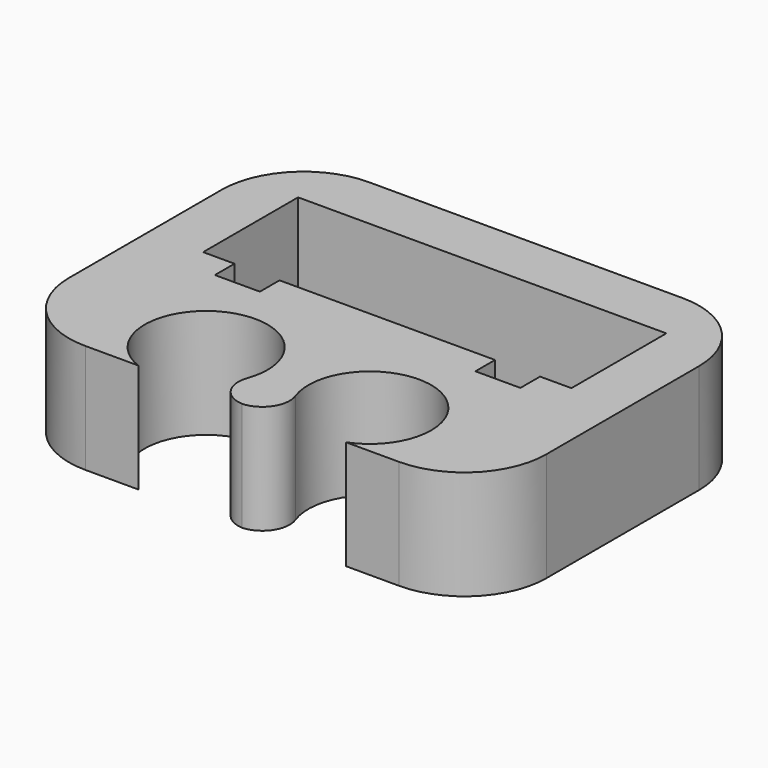
from build123d import *

# Parameters (mm, degrees)
F1_DEPTH    = 4
F2_R        = 3
F3_T1_DEPTH = 15.252055078


# Not quite as in the source:
# - a fillet or chamfer that OpenCascade refuses, or shapes differently, is made with other operations: its cross-section is extruded or revolved along the edge and cut away or added


with BuildPart() as f1:
    # F0 (on Top) → F1 (new body)
    with BuildSketch(Plane.XY):
        with BuildLine():
            Line((8.75, 4.175), (-8.75, 4.175))
            Line((-8.75, 4.175), (-8.75, -8.825))
            Line((-8.75, -8.825), (-3.8077747211, -8.825))
            ThreePointArc((-3.8077747211, -8.825), (-4.2737752701, -4.8702772279), (-0.75, -6.725))
            ThreePointArc((-0.75, -6.725), (-1.1452772279, -7.9987752701), (-2.1922252789, -8.825))
            Line((-2.1922252789, -8.825), (2.1922252789, -8.825))
            ThreePointArc((2.1922252789, -8.825), (1.7262247299, -4.8702772279), (5.25, -6.725))
            ThreePointArc((5.25, -6.725), (4.8547227721, -7.9987752701), (3.8077747211, -8.825))
            Line((3.8077747211, -8.825), (8.75, -8.825))
            Line((8.75, -8.825), (8.75, 4.175))
        make_face()
        Polygon((-6.75, 2.175), (6.75, 2.175), (6.75, -2.175), (5.6, -2.175), (5.6, -3.075), (3.95, -3.075), (3.95, -2.175), (-3.95, -2.175), (-3.95, -3.075), (-5.6, -3.075), (-5.6, -2.175), (-6.75, -2.175), align=None, mode=Mode.SUBTRACT)
    extrude(amount=F1_DEPTH)

    # F2
    f2_edges = [f1.edges().sort_by_distance(p)[0] for p in [
        (-8.75, 4.175, 2),
        (-8.75, -8.825, 2),
        (8.75, -8.825, 2),
        (8.75, 4.175, 2),
    ]]
    fillet(f2_edges, radius=F2_R)

    # F3: fillet of radius 1 on 2 edges, made by hand

    # F3_s2 → F3_t1 (cut)
    with BuildSketch(Plane.XY.offset(-5.626027539)):
        with BuildLine():
            ThreePointArc((0.88279449, -7.4865384615), (0.7598795231, -8.4001254044), (-0.0581857367, -8.825))
            Line((-0.0581857367, -8.825), (2.1922252789, -8.825))
            ThreePointArc((2.1922252789, -8.825), (1.3916632316, -8.2984525222), (0.88279449, -7.4865384615))
        make_face()
        with BuildLine():
            ThreePointArc((0.0581857367, -8.825), (-0.7598795231, -8.4001254044), (-0.88279449, -7.4865384615))
            ThreePointArc((-0.88279449, -7.4865384615), (-1.3916632316, -8.2984525222), (-2.1922252789, -8.825))
            Line((-2.1922252789, -8.825), (0.0581857367, -8.825))
        make_face()
    extrude(amount=F3_T1_DEPTH, mode=Mode.SUBTRACT)


solid = f1.part
